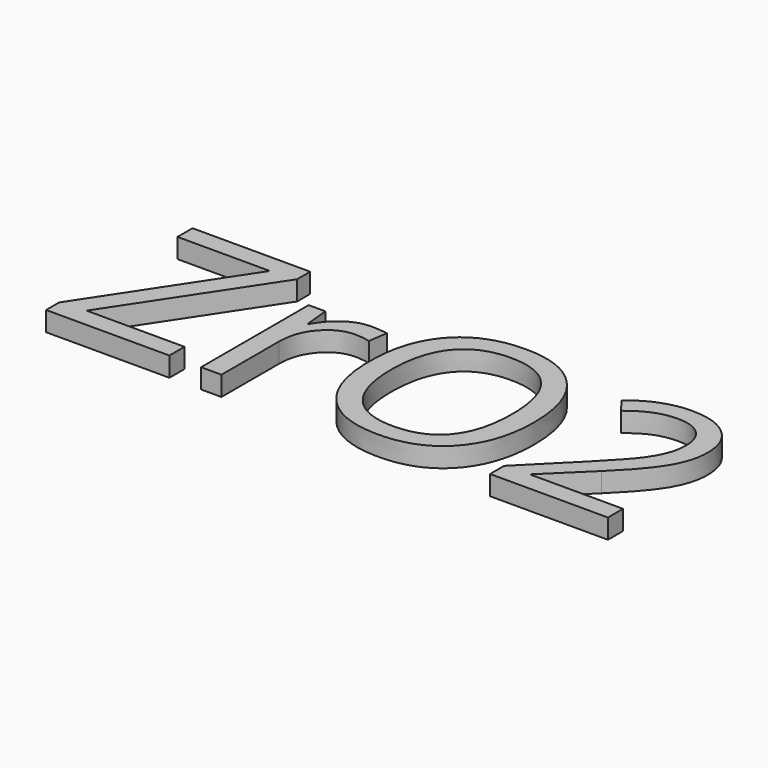
from build123d import *

# Parameters (mm, degrees)
F0_TEXT_SIZE = 12.8162338963
F1_DEPTH     = 1


# Not quite as in the source:
# - Text() gives the source's letters only with a copy of the font that has no kerning and outlines rounded to 1/6400 em; it was checked with that copy


with BuildPart() as f1:
    # F0 (on Top) → F1 (new body)
    with BuildSketch(Plane.XY):
        with Locations((-14.6318428734, -3.7461367093)):
            Text('ZrO2', F0_TEXT_SIZE, font='Open Sans', text_align=(TextAlign.LEFT, TextAlign.BOTTOM))
    extrude(amount=F1_DEPTH)


solid = f1.part
